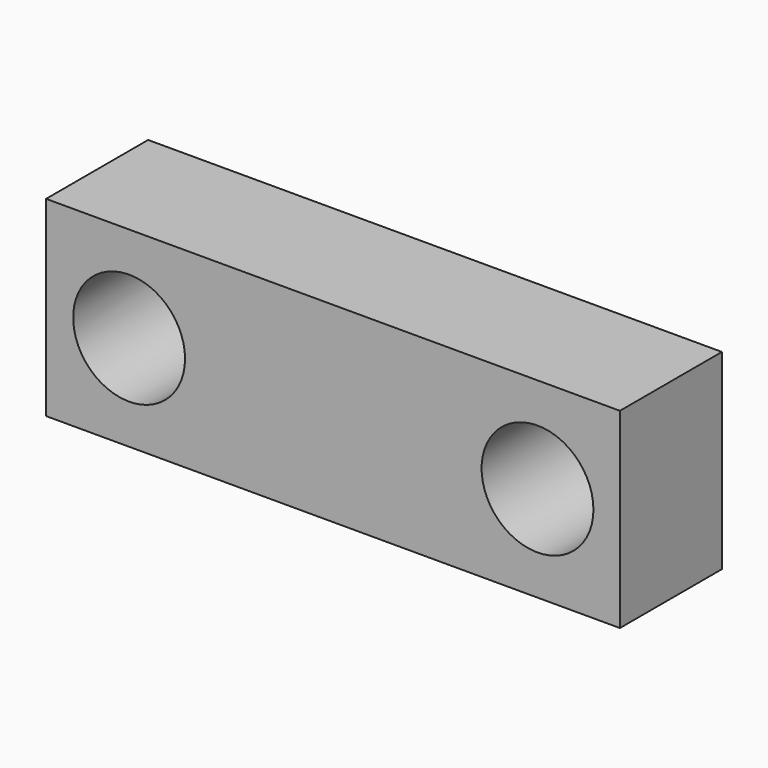
from build123d import *

# Parameters (mm, degrees)
F1_W     = 114.3
F1_H     = 38.1
F1_R     = 11.1418506757
F1_R_2   = 11.1379
F3_DEPTH = 12.7


# Not quite as in the source:
# - the program builds the solid bodies; features that only make, move or delete a surface that nothing else refers to are left out


with BuildPart() as f3:
    # F1 (on face) → F3 (new body, symmetric)
    with BuildSketch(Plane.XZ):
        Rectangle(F1_W, F1_H)
        with Locations((-40.6111367047, 0)):
            Circle(F1_R, mode=Mode.SUBTRACT)
        with Locations((40.7379063194, 0)):
            Circle(F1_R_2, mode=Mode.SUBTRACT)
    extrude(amount=F3_DEPTH, both=True)


solid = f3.part
